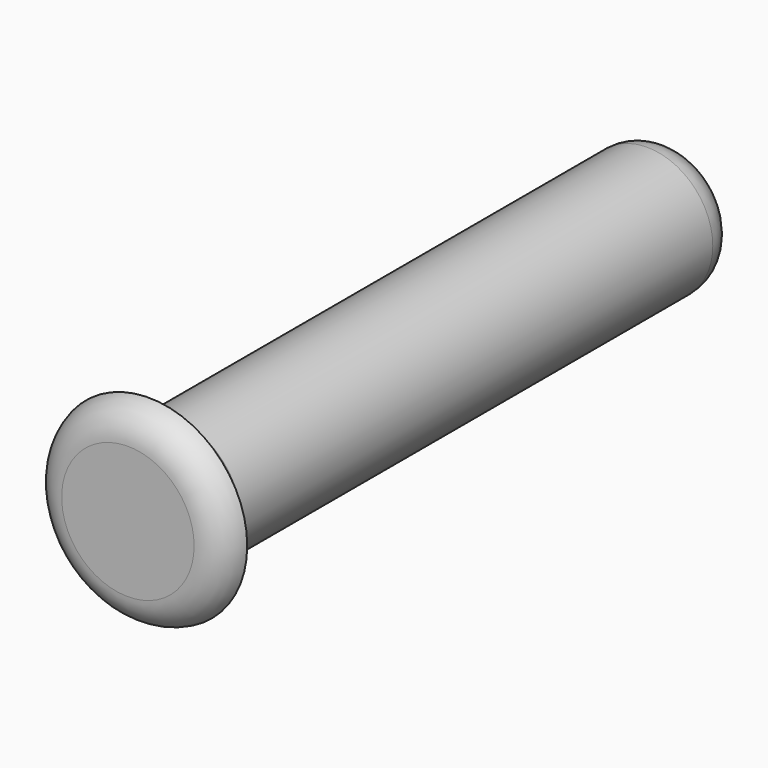
from build123d import *

# Parameters (mm, degrees)
F0_R     = 10
F1_DEPTH = 104
F2_R     = 15
F3_DEPTH = 4
F4_R     = 4.99999


# Not quite as in the source:
# - a fillet or chamfer that OpenCascade refuses, or shapes differently, is made with other operations: its cross-section is extruded or revolved along the edge and cut away or added
# - a fillet or chamfer is up to 0.001 mm smaller than in the source, because OpenCascade refuses the exact size


with BuildPart() as f1:
    # F0 (on Front) → F1 (new body)
    with BuildSketch(Plane.XZ):
        Circle(F0_R)
    extrude(amount=F1_DEPTH)

    # F2 (on face) → F3 (join)
    with BuildSketch(Plane.XZ.offset(104)):
        Circle(F2_R)
    extrude(amount=-F3_DEPTH)

    # F4 (radius 5 in the source; OpenCascade refuses exactly that, so slightly less here)
    f4_edges = [f1.edges().sort_by_distance(p)[0] for p in [
        (-10, -100, 0),
    ]]
    fillet(f4_edges, radius=F4_R)

    # F5: fillet of radius 5 on 2 edges, made by hand

    # F5_s1 → F5_t2 (revolve, cut)
    with BuildSketch(Plane.XY):
        with BuildLine():
            ThreePointArc((15, -100), (13.2632981746, -102.8729833462), (10.1010205144, -104))
            Line((10.1010205144, -104), (15, -104))
            Line((15, -104), (15, -100))
        make_face()
    revolve(axis=Axis((0, -104, 0), (0, -1, 0)), mode=Mode.SUBTRACT)

    # F5_s3 → F5_t4 (revolve, cut)
    with BuildSketch(Plane.XY):
        with BuildLine():
            ThreePointArc((10, -5), (8.5355339059, -1.4644660941), (5, 0))
            Line((5, 0), (10, 0))
            Line((10, 0), (10, -5))
        make_face()
    revolve(axis=Axis((0, 0, 0), (0, -1, 0)), mode=Mode.SUBTRACT)


solid = f1.part
